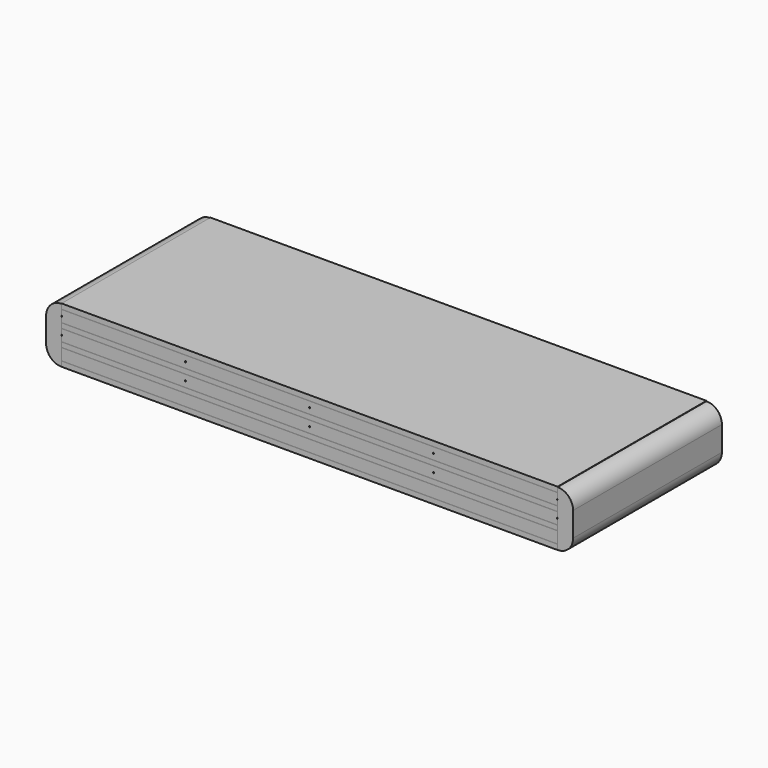
from build123d import *

# Parameters (mm, degrees)
F0_W           = 203.2
F0_H           = 0.1524
F1_DEPTH       = 76.2
F0_H_2         = 1.905
F2_DEPTH       = 76.2
F0_H_3         = 4.6736
F3_DEPTH       = 76.2
F4_W           = 76.2
F4_H           = 22.7076
F5_DEPTH       = 6.35
F6_W           = 76.2
F6_H           = 22.7076
F7_DEPTH       = 6.35
F8_R           = 0.254
F9_DEPTH       = 38.1
F10_R          = 0.254
F11_DEPTH      = 38.1
F12_T1_DEPTH   = 107.95
F12_T3_DEPTH   = 107.95
F12_2_T1_DEPTH = 107.95
F12_2_T3_DEPTH = 107.95
F13_DEPTH      = 25.4
F14_DEPTH      = 25.4
F15_R          = 0.254
F16_R          = 0.254
F17_DEPTH      = 25.4
F18_DEPTH      = 38.1


# Not quite as in the source:
# - a fillet or chamfer that OpenCascade refuses, or shapes differently, is made with other operations: its cross-section is extruded or revolved along the edge and cut away or added


with BuildPart() as f1:
    # F0 (on Front) → F1 (new body)
    with BuildSketch(Plane.XZ):
        with Locations((60.8575803399, -11.7442150349)):
            Rectangle(F0_W, F0_H)
    extrude(amount=F1_DEPTH)


with BuildPart() as f1b:
    # F0 (on Front) → F1, piece 2 (new body)
    with BuildSketch(Plane.XZ):
        with Locations((60.8575803399, -9.6868150349)):
            Rectangle(F0_W, F0_H)
    extrude(amount=F1_DEPTH)


with BuildPart() as f1c:
    # F0 (on Front) → F1, piece 3 (new body)
    with BuildSketch(Plane.XZ):
        with Locations((60.8575803399, -4.8608150349)):
            Rectangle(F0_W, F0_H)
    extrude(amount=F1_DEPTH)


with BuildPart() as f1d:
    # F0 (on Front) → F1, piece 4 (new body)
    with BuildSketch(Plane.XZ):
        with Locations((60.8575803399, -2.8034150349)):
            Rectangle(F0_W, F0_H)
    extrude(amount=F1_DEPTH)


with BuildPart() as f1e:
    # F0 (on Front) → F1, piece 5 (new body)
    with BuildSketch(Plane.XZ):
        with Locations((60.8575803399, 2.0225849651)):
            Rectangle(F0_W, F0_H)
    extrude(amount=F1_DEPTH)


with BuildPart() as f1f:
    # F0 (on Front) → F1, piece 6 (new body)
    with BuildSketch(Plane.XZ):
        with Locations((60.8575803399, 4.0799849651)):
            Rectangle(F0_W, F0_H)
    extrude(amount=F1_DEPTH)


with BuildPart() as f1g:
    # F0 (on Front) → F1, piece 7 (new body)
    with BuildSketch(Plane.XZ):
        with Locations((60.8575803399, 8.9059849651)):
            Rectangle(F0_W, F0_H)
    extrude(amount=F1_DEPTH)


with BuildPart() as f1h:
    # F0 (on Front) → F1, piece 8 (new body)
    with BuildSketch(Plane.XZ):
        with Locations((60.8575803399, 10.9633849651)):
            Rectangle(F0_W, F0_H)
    extrude(amount=F1_DEPTH)


with BuildPart() as f2:
    # F0 (on Front) → F2 (new body)
    with BuildSketch(Plane.XZ):
        with Locations((60.8575803399, -10.7155150349)):
            Rectangle(F0_W, F0_H_2)
    extrude(amount=F2_DEPTH)


with BuildPart() as f2b:
    # F0 (on Front) → F2, piece 2 (new body)
    with BuildSketch(Plane.XZ):
        with Locations((60.8575803399, -3.8321150349)):
            Rectangle(F0_W, F0_H_2)
    extrude(amount=F2_DEPTH)


with BuildPart() as f2c:
    # F0 (on Front) → F2, piece 3 (new body)
    with BuildSketch(Plane.XZ):
        with Locations((60.8575803399, 3.0512849651)):
            Rectangle(F0_W, F0_H_2)
    extrude(amount=F2_DEPTH)


with BuildPart() as f2d:
    # F0 (on Front) → F2, piece 4 (new body)
    with BuildSketch(Plane.XZ):
        with Locations((60.8575803399, 9.9346849651)):
            Rectangle(F0_W, F0_H_2)
    extrude(amount=F2_DEPTH)


with BuildPart() as f3:
    # F0 (on Front) → F3 (new body)
    with BuildSketch(Plane.XZ):
        with Locations((60.8575803399, 6.4929849651)):
            Rectangle(F0_W, F0_H_3)
    extrude(amount=F3_DEPTH)

    # F10 (on face) → F11 (cut)
    with BuildSketch(Plane.XZ.offset(76.2)):
        with BuildLine():
            ThreePointArc((-40.7424196601, 6.2389849651), (-40.5628145377, 6.3133798427), (-40.4884196601, 6.4929849651))
            ThreePointArc((-40.4884196601, 6.4929849651), (-40.5628145377, 6.6725900875), (-40.7424196601, 6.7469849651))
            Line((-40.7424196601, 6.7469849651), (-40.7424196601, 6.2389849651))
        make_face()
        with BuildLine():
            Line((-40.7424196601, 6.2389849651), (-40.7424196601, 6.7469849651))
            ThreePointArc((-40.7424196601, 6.7469849651), (-40.9964196601, 6.4929849651), (-40.7424196601, 6.2389849651))
        make_face()
        with BuildLine():
            Line((162.4575803399, 6.1543183082), (162.4575803399, 6.6623182886))
            ThreePointArc((162.4575803399, 6.6623182886), (162.2035097843, 6.4083182984), (162.4575803399, 6.1543183082))
        make_face()
        with Locations((60.8575803399, 6.4929849651)):
            Circle(F10_R)
    extrude(amount=-F11_DEPTH, mode=Mode.SUBTRACT)

    # F10 (on face) → F14 (cut)
    with BuildSketch(Plane.XZ.offset(76.2)):
        with Locations((10.0575803399, 6.4929849651)):
            Circle(F10_R)
        with Locations((111.6575803399, 6.4929849651)):
            Circle(F10_R)
    extrude(amount=-F14_DEPTH, mode=Mode.SUBTRACT)


with BuildPart() as f3b:
    # F0 (on Front) → F3, piece 2 (new body)
    with BuildSketch(Plane.XZ):
        with Locations((60.8575803399, -0.3904150349)):
            Rectangle(F0_W, F0_H_3)
    extrude(amount=F3_DEPTH)

    # F8 (on face) → F9 (cut)
    with BuildSketch(Plane.XZ.offset(76.2)):
        with BuildLine():
            ThreePointArc((-40.7424196601, -0.6444150349), (-40.5628145377, -0.5700201573), (-40.4884196601, -0.3904150349))
            ThreePointArc((-40.4884196601, -0.3904150349), (-40.5628145377, -0.2108099125), (-40.7424196601, -0.1364150349))
            Line((-40.7424196601, -0.1364150349), (-40.7424196601, -0.6444150349))
        make_face()
        with BuildLine():
            Line((-40.7424196601, -0.6444150349), (-40.7424196601, -0.1364150349))
            ThreePointArc((-40.7424196601, -0.1364150349), (-40.9964196601, -0.3904150349), (-40.7424196601, -0.6444150349))
        make_face()
        with BuildLine():
            Line((162.4575803399, -0.6444150349), (162.4575803399, -0.1364150349))
            ThreePointArc((162.4575803399, -0.1364150349), (162.2035803399, -0.3904150349), (162.4575803399, -0.6444150349))
        make_face()
        with Locations((60.8575803399, -0.3904150349)):
            Circle(F8_R)
    extrude(amount=-F9_DEPTH, mode=Mode.SUBTRACT)

    # F8 (on face) → F13 (cut)
    with BuildSketch(Plane.XZ.offset(76.2)):
        with Locations((10.0575803399, -0.3904150349)):
            Circle(F8_R)
        with Locations((111.6575803399, -0.3904150349)):
            Circle(F8_R)
    extrude(amount=-F13_DEPTH, mode=Mode.SUBTRACT)


with BuildPart() as f3c:
    # F0 (on Front) → F3, piece 3 (new body)
    with BuildSketch(Plane.XZ):
        with Locations((60.8575803399, -7.2738150349)):
            Rectangle(F0_W, F0_H_3)
    extrude(amount=F3_DEPTH)


with BuildPart() as f5:
    # F4 (on face) → F5 (new body)
    with BuildSketch(Plane.YZ.offset(162.4575803399)):
        with Locations((-38.1, -0.4666150349)):
            Rectangle(F4_W, F4_H)
    extrude(amount=F5_DEPTH)

    # F12: fillet of radius 6.35 on 4 edges, made by hand

    # F12_s2 → F12_t1 (cut)
    with BuildSketch(Plane.XZ.offset(-15.875)):
        with BuildLine():
            ThreePointArc((162.4575803399, -11.8204150349), (166.9477084004, -9.9605430954), (168.8075803399, -5.4704150349))
            Line((168.8075803399, -5.4704150349), (168.8075803399, -11.8204150349))
            Line((168.8075803399, -11.8204150349), (162.4575803399, -11.8204150349))
        make_face()
    extrude(amount=F12_T1_DEPTH, mode=Mode.SUBTRACT)

    # F12_s4 → F12_t3 (cut)
    with BuildSketch(Plane.XZ.offset(-15.875)):
        with BuildLine():
            ThreePointArc((162.4575803399, 10.8871849651), (166.9477084004, 9.0273130256), (168.8075803399, 4.5371849651))
            Line((168.8075803399, 4.5371849651), (168.8075803399, 10.8871849651))
            Line((168.8075803399, 10.8871849651), (162.4575803399, 10.8871849651))
        make_face()
    extrude(amount=F12_T3_DEPTH, mode=Mode.SUBTRACT)


with BuildPart() as f7:
    # F6 (on face) → F7 (new body)
    with BuildSketch(Plane(origin=(-40.7424196601, 0, 0), x_dir=(0, -1, 0), z_dir=(-1, 0, 0))):
        with Locations((38.1, -0.4666150349)):
            Rectangle(F6_W, F6_H)
    extrude(amount=F7_DEPTH)

    # F12#2: fillet of radius 6.35 on 4 edges, made by hand

    # F12_2_s2 → F12_2_t1 (cut)
    with BuildSketch(Plane.XZ.offset(-15.875)):
        with BuildLine():
            ThreePointArc((-40.7424196601, 10.8871849651), (-45.2325477206, 9.0273130256), (-47.0924196601, 4.5371849651))
            Line((-47.0924196601, 4.5371849651), (-47.0924196601, 10.8871849651))
            Line((-47.0924196601, 10.8871849651), (-40.7424196601, 10.8871849651))
        make_face()
    extrude(amount=F12_2_T1_DEPTH, mode=Mode.SUBTRACT)

    # F12_2_s4 → F12_2_t3 (cut)
    with BuildSketch(Plane.XZ.offset(-15.875)):
        with BuildLine():
            ThreePointArc((-47.0924196601, -5.4704150349), (-45.2325477206, -9.9605430954), (-40.7424196601, -11.8204150349))
            Line((-40.7424196601, -11.8204150349), (-47.0924196601, -11.8204150349))
            Line((-47.0924196601, -11.8204150349), (-47.0924196601, -5.4704150349))
        make_face()
    extrude(amount=F12_2_T3_DEPTH, mode=Mode.SUBTRACT)


with BuildPart() as f17_tool:
    # F15 (on face) + F16 (on face) → F17 (new body)
    with BuildSketch(Plane(origin=(0, 0, 0), x_dir=(-1, 0, 0), z_dir=(0, 1, 0))):
        with Locations((-111.6575803399, 6.4929849651)):
            Circle(F15_R)
        with Locations((-10.0575803399, 6.4929849651)):
            Circle(F15_R)
    with BuildSketch(Plane(origin=(0, 0, 0), x_dir=(-1, 0, 0), z_dir=(0, 1, 0))):
        with Locations((-111.6575803399, -0.3904150349)):
            Circle(F16_R)
        with Locations((-10.0575803399, -0.3904150349)):
            Circle(F16_R)
    extrude(amount=-F17_DEPTH)


with BuildPart() as f3_1:
    add(f3.part)

    # F17: cut by f17_tool
    add(f17_tool.part, mode=Mode.SUBTRACT)


with BuildPart() as f3b_1:
    add(f3b.part)

    # F17: cut by f17_tool
    add(f17_tool.part, mode=Mode.SUBTRACT)


with BuildPart() as f18_tool:
    # F16 (on face) + F15 (on face) → F18 (new body)
    with BuildSketch(Plane(origin=(0, 0, 0), x_dir=(-1, 0, 0), z_dir=(0, 1, 0))):
        with Locations((-62.1275803399, -0.3904150349)):
            Circle(F16_R)
        with Locations((-59.5875803399, -0.3904150349)):
            Circle(F16_R)
    with BuildSketch(Plane(origin=(0, 0, 0), x_dir=(-1, 0, 0), z_dir=(0, 1, 0))):
        with Locations((-62.1275803399, 6.4929849651)):
            Circle(F15_R)
        with Locations((-59.5875803399, 6.4929849651)):
            Circle(F15_R)
    extrude(amount=-F18_DEPTH)


with BuildPart() as f3_2:
    add(f3_1.part)

    # F18: cut by f18_tool
    add(f18_tool.part, mode=Mode.SUBTRACT)


with BuildPart() as f3b_2:
    add(f3b_1.part)

    # F18: cut by f18_tool
    add(f18_tool.part, mode=Mode.SUBTRACT)


solid = Compound([f1.part, f1b.part, f1c.part, f1d.part, f1e.part, f1f.part, f1g.part, f1h.part, f2.part, f2b.part, f2c.part, f2d.part, f3c.part, f5.part, f7.part, f3_2.part, f3b_2.part])
